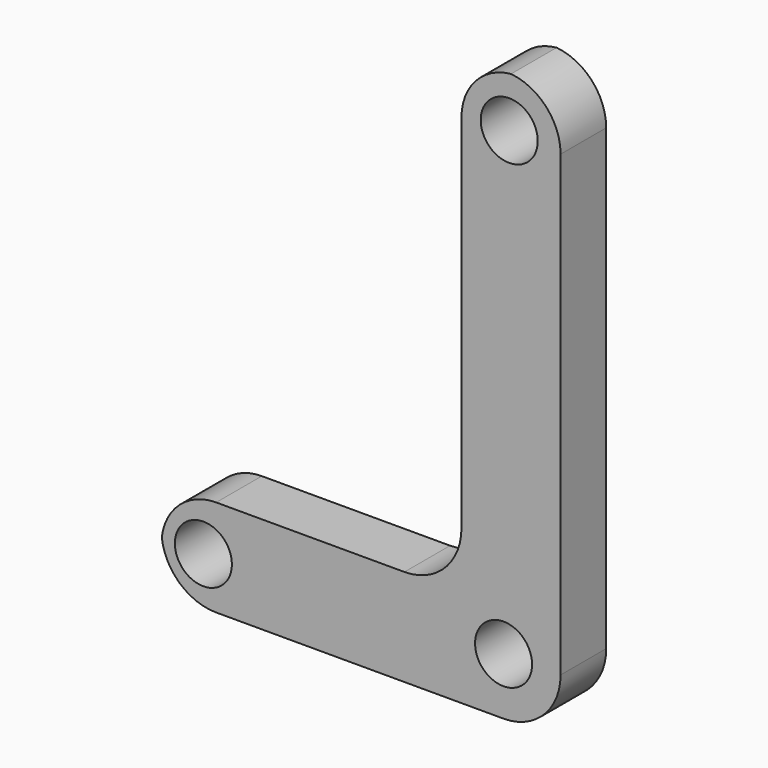
from build123d import *

# Parameters (mm, degrees)
F0_R        = 3.175
F1_DEPTH    = 6.35
F2_T1_DEPTH = 36.83
F3_T1_DEPTH = 36.83


# Not quite as in the source:
# - a fillet or chamfer that OpenCascade refuses, or shapes differently, is made with other operations: its cross-section is extruded or revolved along the edge and cut away or added


with BuildPart() as f1:
    # F0 (on Front) → F1 (new body)
    with BuildSketch(Plane.XZ):
        with BuildLine():
            Line((11.0398714598, -22.7022875817), (11.0398714598, 34.4477124183))
            Line((11.0398714598, 34.4477124183), (0, 34.4477124183))
            Line((0, 34.4477124183), (0, -11.9114368191))
            ThreePointArc((0, -11.9114368191), (-1.8598719395, -16.4015648796), (-6.35, -18.2614368191))
            Line((-6.35, -18.2614368191), (-33.4101285402, -18.2614368191))
            Line((-33.4101285402, -18.2614368191), (-33.4101285402, -29.0522875817))
            Line((-33.4101285402, -29.0522875817), (4.6898714598, -29.0522875817))
            ThreePointArc((4.6898714598, -29.0522875817), (9.1799995204, -27.1924156422), (11.0398714598, -22.7022875817))
        make_face()
        with Locations((-28.7397336215, -23.7723737955)):
            Circle(F0_R, mode=Mode.SUBTRACT)
        with Locations((4.6898714598, -22.7022875817)):
            Circle(F0_R, mode=Mode.SUBTRACT)
        with Locations((5.3221737035, 28.8079940212)):
            Circle(F0_R, mode=Mode.SUBTRACT)
    extrude(amount=F1_DEPTH)

    # F2: fillet of radius 6.096 on 2 edges, made by hand

    # F2_s2 → F2_t1 (cut)
    with BuildSketch(Plane.XZ.offset(-15.24)):
        with BuildLine():
            ThreePointArc((-27.3141285402, -18.2614368191), (-31.6246514783, -20.046913881), (-33.4101285402, -24.3574368191))
            Line((-33.4101285402, -24.3574368191), (-33.4101285402, -18.2614368191))
            Line((-33.4101285402, -18.2614368191), (-27.3141285402, -18.2614368191))
        make_face()
        with BuildLine():
            ThreePointArc((-33.4101285402, -22.9562875817), (-31.6246514783, -27.2668105198), (-27.3141285402, -29.0522875817))
            Line((-27.3141285402, -29.0522875817), (-33.4101285402, -29.0522875817))
            Line((-33.4101285402, -29.0522875817), (-33.4101285402, -22.9562875817))
        make_face()
    extrude(amount=F2_T1_DEPTH, mode=Mode.SUBTRACT)

    # F3: fillet of radius 6.096 on 2 edges, made by hand

    # F3_s2 → F3_t1 (cut)
    with BuildSketch(Plane.XZ.offset(-15.24)):
        with BuildLine():
            ThreePointArc((6.096, 34.4477124183), (1.7854770619, 32.6622353564), (0, 28.3517124183))
            Line((0, 28.3517124183), (0, 34.4477124183))
            Line((0, 34.4477124183), (6.096, 34.4477124183))
        make_face()
        with BuildLine():
            ThreePointArc((11.0398714598, 28.3517124183), (9.2543943979, 32.6622353564), (4.9438714598, 34.4477124183))
            Line((4.9438714598, 34.4477124183), (11.0398714598, 34.4477124183))
            Line((11.0398714598, 34.4477124183), (11.0398714598, 28.3517124183))
        make_face()
    extrude(amount=F3_T1_DEPTH, mode=Mode.SUBTRACT)


solid = f1.part
